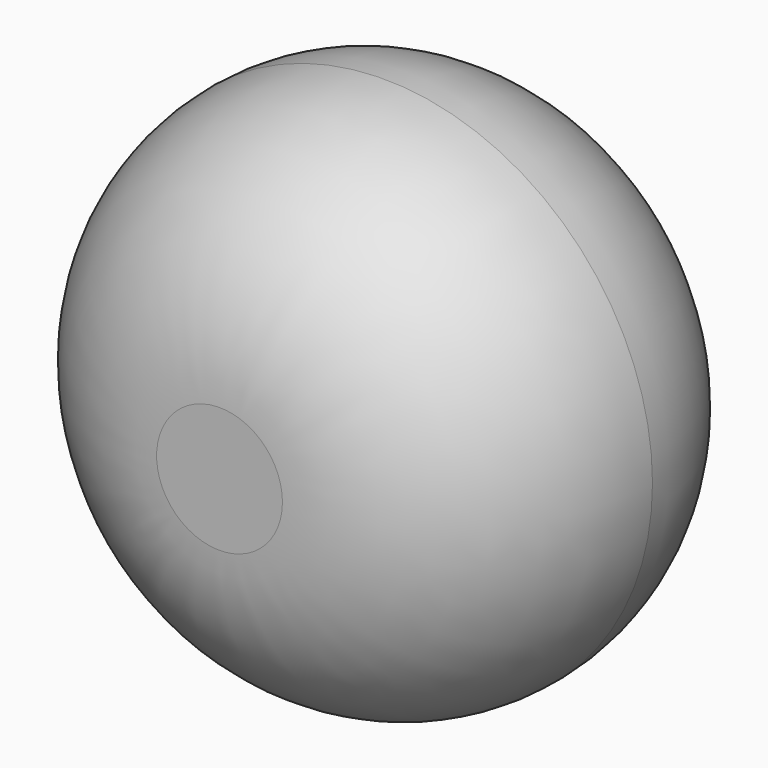
from build123d import *

# Parameters (mm, degrees)
F0_R     = 3.2650243754
F1_DEPTH = 5
F2_R     = 2.49999


# Not quite as in the source:
# - a fillet or chamfer is up to 0.001 mm smaller than in the source, because OpenCascade refuses the exact size


with BuildPart() as f1:
    # F0 (on Front) → F1 (new body)
    with BuildSketch(Plane.XZ):
        Circle(F0_R)
    extrude(amount=F1_DEPTH)

    # F2 (radius 2.5 in the source; OpenCascade refuses exactly that, so slightly less here)
    f2_edges = [f1.edges().sort_by_distance(p)[0] for p in [
        (-3.265024, -5, 0),
        (-3.265024, 0, 0),
    ]]
    fillet(f2_edges, radius=F2_R)


solid = f1.part
